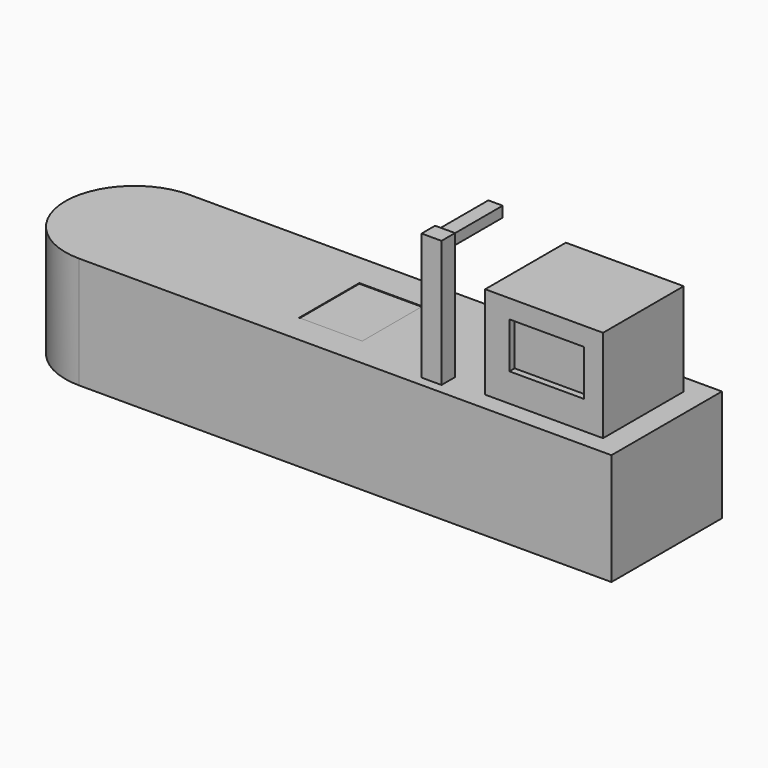
from build123d import *

# Parameters (mm, degrees)
F1_DEPTH  = 1041.6941642761
F2_W      = 1126.0592937469
F2_H      = 963.8655930758
F3_DEPTH  = 912.1903181076
F4_W      = 1126.0592937469
F4_H      = 963.8655930758
F5_DEPTH  = 25.4
F7_W      = 516.755759716
F7_H      = 380.2199363708
F8_DEPTH  = 0.79375
F9_DEPTH  = 49.5742298663
F10_W     = 748.920917511
F10_H     = 427.7250766754
F11_DEPTH = 62.6353546977
F12_W     = 712.7413749695
F12_H     = 437.5553131104
F13_DEPTH = 62.6364
F14_W     = 602.8727293015
F14_H     = 718.7194526196
F15_DEPTH = 6.35
F16_W     = 190.1788711548
F16_H     = 161.4509820938
F17_DEPTH = 1212.1773958206
F18_W     = 137.4664306641
F18_H     = 100.9991168976
F19_DEPTH = 605.9129238129


# Not quite as in the source:
# - a length typed as a fraction of an inch, garbled in the dataset ("3 / 203.2 mm" for 3/8 in), is restored


with BuildPart() as f1:
    # F0 (on Top) → F1 (new body)
    with BuildSketch(Plane.XY):
        with BuildLine():
            Line((1275.3586769104, 60.9520673752), (0, 60.9520673752))
            ThreePointArc((0, 60.9520673752), (-659.7163081169, -598.7642407417), (0, -1258.4805488586))
            Line((0, -1258.4805488586), (5085.4144096375, -1258.4805488586))
            Line((5085.4144096375, -1258.4805488586), (5085.4144096375, 60.9520673752))
            Line((5085.4144096375, 60.9520673752), (1275.3586769104, 60.9520673752))
        make_face()
    extrude(amount=F1_DEPTH)

    # F2 (on face) → F3 (join)
    with BuildSketch(Plane.XY.offset(1041.6941642761)):
        with Locations((4301.8175363541, -601.2575253844)):
            Rectangle(F2_W, F2_H)
    extrude(amount=F3_DEPTH)

    # F4 (on face) → F5 (join)
    with BuildSketch(Plane.XY.offset(1041.6941642761)):
        with BuildLine():
            Line((5085.4144096375, -1258.4805488586), (5085.4144096375, 60.9520673752))
            Line((5085.4144096375, 60.9520673752), (0, 60.9520673752))
            ThreePointArc((0, 60.9520673752), (-659.7163081169, -598.7642407417), (0, -1258.4805488586))
            Line((0, -1258.4805488586), (5085.4144096375, -1258.4805488586))
        make_face()
        with Locations((4301.8175363541, -601.2575253844)):
            Rectangle(F4_W, F4_H, mode=Mode.SUBTRACT)
    extrude(amount=F5_DEPTH)

    # F7 (on face) → F8 (cut)
    with BuildSketch(Plane(origin=(3738.7878894806, 0, 0), x_dir=(0, -1, 0), z_dir=(-1, 0, 0))):
        with Locations((570.4796612263, 1562.8325939178)):
            Rectangle(F7_W, F7_H)
    extrude(amount=-F8_DEPTH, mode=Mode.SUBTRACT)

    # F7 (on face) → F9 (cut)
    with BuildSketch(Plane(origin=(3738.7878894806, 0, 0), x_dir=(0, -1, 0), z_dir=(-1, 0, 0))):
        with Locations((570.4796612263, 1562.8325939178)):
            Rectangle(F7_W, F7_H)
    extrude(amount=-F9_DEPTH, mode=Mode.SUBTRACT)

    # F10 (on face) → F11 (cut)
    with BuildSketch(Plane(origin=(0, -119.3247288465, 0), x_dir=(-1, 0, 0), z_dir=(0, 1, 0))):
        with Locations((-4334.9487781525, 1559.3398809433)):
            Rectangle(F10_W, F10_H)
    extrude(amount=-F11_DEPTH, mode=Mode.SUBTRACT)

    # F12 (on face) → F13 (cut)
    with BuildSketch(Plane.XZ.offset(1083.1903219223)):
        with Locations((4326.6184329987, 1557.3492050171)):
            Rectangle(F12_W, F12_H)
    extrude(amount=-F13_DEPTH, mode=Mode.SUBTRACT)

    # F14 (on face) → F15 (cut)
    with BuildSketch(Plane.XY.offset(1067.0941642761)):
        with Locations((2180.1822781563, -620.3462034464)):
            Rectangle(F14_W, F14_H)
    extrude(amount=-F15_DEPTH, mode=Mode.SUBTRACT)

    # F16 (on face) → F17 (join)
    with BuildSketch(Plane.XY.offset(1067.0941642761)):
        with Locations((3291.446685791, -1083.8199257851)):
            Rectangle(F16_W, F16_H)
    extrude(amount=F17_DEPTH)

    # F18 (on face) → F19 (join)
    with BuildSketch(Plane(origin=(0, -1003.0944347382, 0), x_dir=(-1, 0, 0), z_dir=(0, 1, 0))):
        with Locations((-3288.6855602264, 2203.5087347031)):
            Rectangle(F18_W, F18_H)
    extrude(amount=F19_DEPTH)


solid = f1.part
